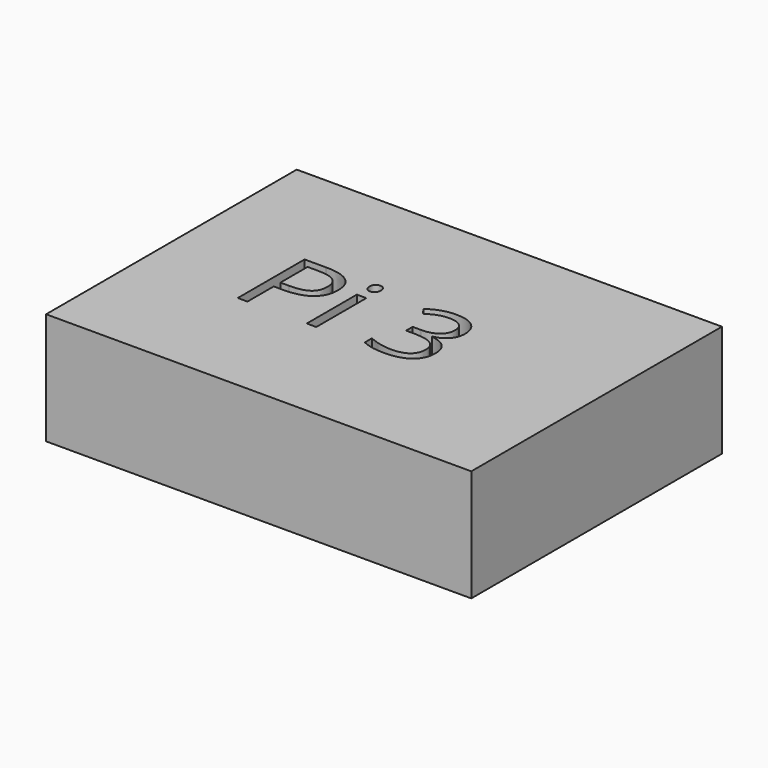
from build123d import *

# Parameters (mm, degrees)
F0_W         = 95
F0_H         = 70
F1_DEPTH     = 25
F2_TEXT_SIZE = 26.1441028366
F3_DEPTH     = 25


# Not quite as in the source:
# - Text() gives the source's letters only with a copy of the font that has no kerning and outlines rounded to 1/6400 em; it was checked with that copy


with BuildPart() as f1:
    # F0 (on Top) → F1 (new body)
    with BuildSketch(Plane.XY):
        with Locations((-47.5, -35)):
            Rectangle(F0_W, F0_H)
    extrude(amount=F1_DEPTH)

    # F2 (on face) → F3 (cut)
    with BuildSketch(Plane.XY.offset(25)):
        with Locations((-75.2874463797, -44.319216162)):
            Text('Pi 3', F2_TEXT_SIZE, font='Open Sans', text_align=(TextAlign.LEFT, TextAlign.BOTTOM))
    extrude(amount=-F3_DEPTH, mode=Mode.SUBTRACT)


solid = f1.part
